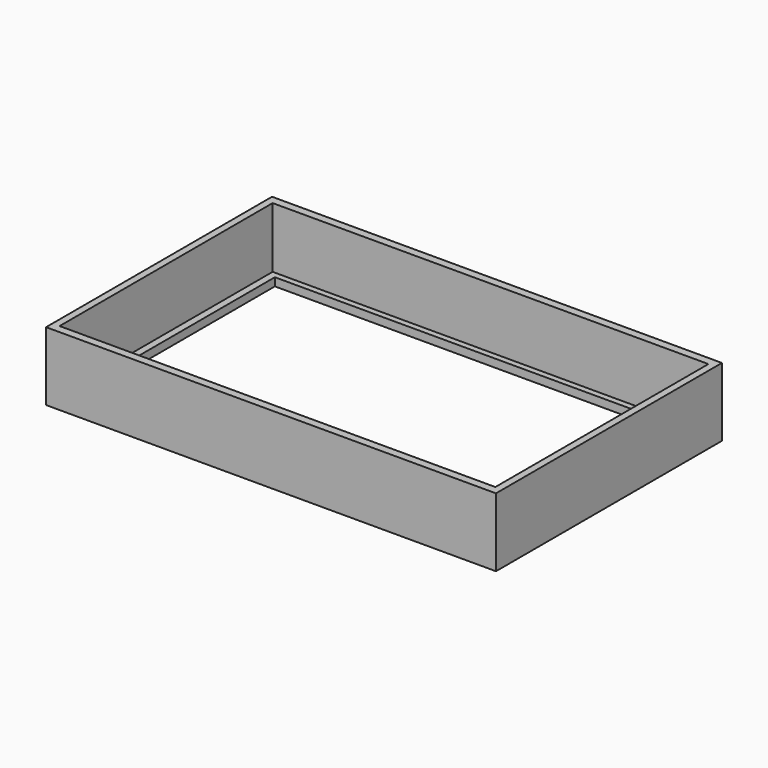
from build123d import *

# Parameters (mm, degrees)
F0_W     = 111.5
F0_H     = 70
F1_DEPTH = 17
F2_W     = 108
F2_H     = 66
F3_DEPTH = 15
F4_W     = 104.5
F4_H     = 63
F5_DEPTH = 17.001


# Not quite as in the source:
# - a feature of the source that left no trace in its solid (it failed there, or was rolled back) is left out


with BuildPart() as f1:
    # F0 (on Top) → F1 (new body)
    with BuildSketch(Plane.XY):
        with Locations((55.75, 35)):
            Rectangle(F0_W, F0_H)
    extrude(amount=F1_DEPTH)

    # F2 (on face) → F3 (cut)
    with BuildSketch(Plane.XY.offset(17)):
        with Locations((55.75, 35)):
            Rectangle(F2_W, F2_H)
    extrude(amount=-F3_DEPTH, mode=Mode.SUBTRACT)

    # F4 (on face) → F5 (cut, through all)
    with BuildSketch(Plane(origin=(0, 0, 0), x_dir=(1, 0, 0), z_dir=(0, 0, -1))):
        with Locations((55.75, -35)):
            Rectangle(F4_W, F4_H)
    extrude(amount=-F5_DEPTH, mode=Mode.SUBTRACT)


solid = f1.part
